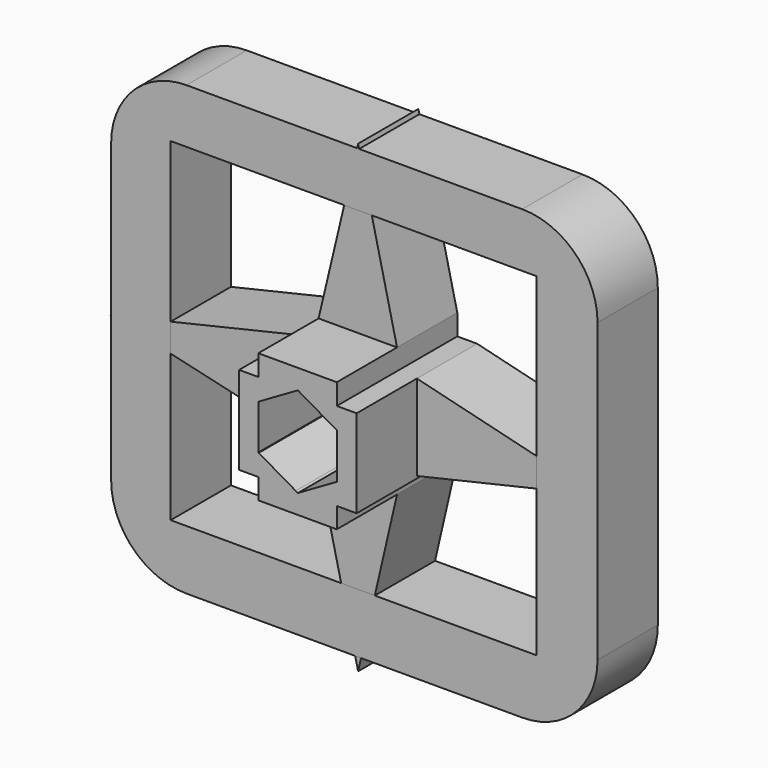
from build123d import *

# Parameters (mm, degrees)
F2_DEPTH = 10
F4_DEPTH = 5
F5_W     = 4.0360325947
F5_H     = 22.1552448347
F5_W_2   = 24.3020709604
F5_H_2   = 3.6066677421
F5_W_3   = 3.9501627907
F5_H_3   = 3.9501599967
F6_DEPTH = 5
F7_R     = 5


with BuildPart() as f2:
    # F1 (on face) → F2 (new body)
    with BuildSketch(Plane.XZ):
        Polygon((-2.6268342044, 2.9277561698), (-2.6268342044, 1.4948317548), (-2.5980762114, 1.4948317548), (-2.5980762114, 1.5), (-0.1251299844, 2.9277561698), align=None)
        Polygon((-2.6268342044, -1.4847409911), (-2.6268342044, 1.4948317548), (-2.6268342044, 2.9277561698), (-3.9005447179, 2.9277561698), (-3.9005447179, -2.9176650569), (-2.6268342044, -2.9176650569), align=None)
        Polygon((-2.6268342044, 4.3151909485), (-2.6268342044, 2.9277561698), (-0.1251299844, 2.9277561698), (0, 3), (0.1251299844, 2.9277561698), (2.5817316491, 2.9277561698), (2.5817316491, 4.3151909485), align=None)
        Polygon((-2.5980762114, -1.4847409911), (-2.6268342044, -1.4847409911), (-2.6268342044, -2.9176650569), (-0.1426083047, -2.9176650569), (-2.5980762114, -1.5), align=None)
        Polygon((2.5980762114, 1.5), (2.5980762114, 1.4948317548), (2.6044766419, 1.4948317548), (2.6044766419, 2.9277561698), (2.5817316491, 2.9277561698), (0.1251299844, 2.9277561698), align=None)
        Polygon((-0.1426083047, -2.9176650569), (-2.6268342044, -2.9176650569), (-2.6268342044, -4.2823553085), (2.5817316491, -4.2823553085), (2.5817316491, -2.9176650569), (0.1426083047, -2.9176650569), (0, -3), align=None)
        Polygon((2.6044766419, 2.9277561698), (2.6044766419, 1.4948317548), (2.6044766419, -2.9176650569), (3.9009321481, -2.9176650569), (3.9009321481, 2.9277561698), align=None)
        Polygon((2.5817316491, -2.9176650569), (2.5817316491, -1.5094365374), (0.1426083047, -2.9176650569), align=None)
    extrude(amount=F2_DEPTH)


with BuildPart() as f4:
    # F3 (on face) → F4 (new body)
    with BuildSketch(Plane(origin=(0, 0, 0), x_dir=(-1, 0, 0), z_dir=(0, 1, 0))):
        Polygon((-3.9009321481, -2.7673800444), (-3.9009321481, 2.9277561698), (-15.8375352621, 0), align=None)
    extrude(amount=-F4_DEPTH)


with BuildPart() as f4b:
    # F3 (on face) → F4, piece 2 (new body)
    with BuildSketch(Plane(origin=(0, 0, 0), x_dir=(-1, 0, 0), z_dir=(0, 1, 0))):
        Polygon((-2.5817316491, 4.3151909485), (0, 4.3151909485), (0, 15.3830023482), align=None)
        Polygon((0, 15.3830023482), (0, 4.3151909485), (2.6268342044, 4.3151909485), align=None)
    extrude(amount=-F4_DEPTH)


with BuildPart() as f4c:
    # F3 (on face) → F4, piece 3 (new body)
    with BuildSketch(Plane(origin=(0, 0, 0), x_dir=(-1, 0, 0), z_dir=(0, 1, 0))):
        Polygon((16.458151862, 0), (3.9005447179, 2.9277561698), (3.9005447179, -2.9176650569), align=None)
    extrude(amount=-F4_DEPTH)


with BuildPart() as f4d:
    # F3 (on face) → F4, piece 4 (new body)
    with BuildSketch(Plane(origin=(0, 0, 0), x_dir=(-1, 0, 0), z_dir=(0, 1, 0))):
        Polygon((0, -15.4520757496), (2.6268342044, -4.2823553085), (-2.5817316491, -4.2823553085), align=None)
    extrude(amount=-F4_DEPTH)


with BuildPart() as f6:
    # F5 (on Front) → F6 (new body)
    with BuildSketch(Plane.XZ):
        with Locations((13.8741279952, 0.4113134928)):
            Rectangle(F5_W, F5_H)
        with Locations((-0.2949237823, 13.2922697812)):
            Rectangle(F5_W_2, F5_H_2)
        Polygon((-16.3961220533, -10.6663089246), (-12.4459592625, -10.6663089246), (-12.4459592625, 11.4889359102), (-12.4459592625, 15.0956036523), (-16.3961220533, 15.0956036523), align=None)
        with Locations((-14.4210406579, -12.6413889229)):
            Rectangle(F5_W_3, F5_H_3)
        with Locations((-0.2949237823, -12.6413889229)):
            Rectangle(F5_W_2, F5_H_3)
        with Locations((13.8741279952, -12.6413889229)):
            Rectangle(F5_W, F5_H_3)
        with Locations((13.8741279952, 13.2922697812)):
            Rectangle(F5_W, F5_H_2)
    extrude(amount=F6_DEPTH)

    # F7
    f7_edges = [f6.edges().sort_by_distance(p)[0] for p in [
        (15.892144, -2.5, -14.616469),
        (-16.396122, -2.5, -14.616469),
        (15.892144, -2.5, 15.095604),
        (-16.396122, -2.5, 15.095604),
    ]]
    fillet(f7_edges, radius=F7_R)


solid = Compound([f2.part, f4.part, f4b.part, f4c.part, f4d.part, f6.part])
